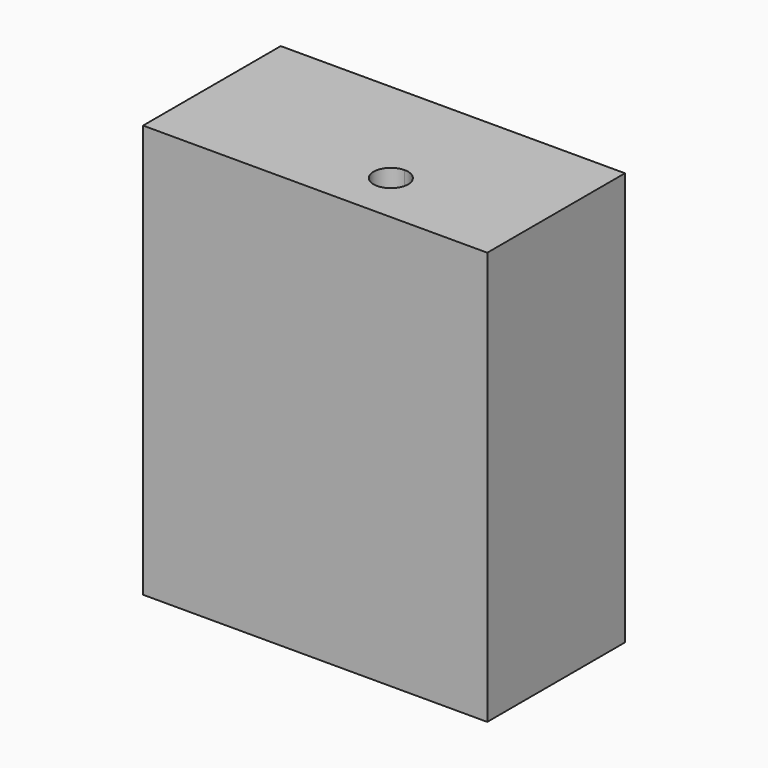
from build123d import *

# Parameters (mm, degrees)
F0_W     = 50
F0_H     = 60
F1_DEPTH = 12.5
F3_DEPTH = 12.5
F5_DEPTH = 60


# Not quite as in the source:
# - a feature names something its author has since deleted; it is built from what else it names


with BuildPart() as f1:
    # F0 (on Front) → F1 (new body, symmetric)
    with BuildSketch(Plane.XZ):
        with Locations((25, 30)):
            Rectangle(F0_W, F0_H)
    extrude(amount=F1_DEPTH, both=True)

    # F2 (on Right) → F3 (cut, symmetric)
    with BuildSketch(Plane.YZ):
        Polygon((-12.1228452772, 60.4202598333), (0, 60.6142282486), (0, 70.6142282486), align=None)
    extrude(amount=F3_DEPTH, both=True, mode=Mode.SUBTRACT)

    # F4 (on Top) → F5 (cut, through all)
    with BuildSketch(Plane.XY):
        with BuildLine():
            ThreePointArc((30, -2.5), (28.232233047, -6.767766953), (32.5, -5))
            ThreePointArc((32.5, -5), (31.767766953, -3.232233047), (30, -2.5))
        make_face()
    extrude(amount=F5_DEPTH, mode=Mode.SUBTRACT)


solid = f1.part
